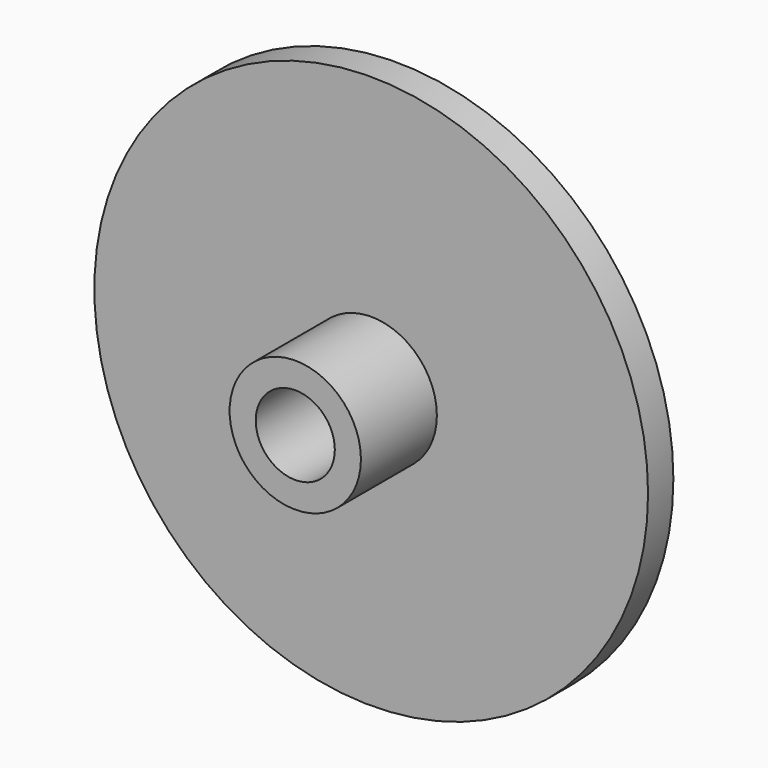
from build123d import *

# Parameters (mm, degrees)
F0_R     = 17.5
F1_DEPTH = 2.00000108
F2_R     = 2.5
F3_DEPTH = 6
F6_DEPTH = 8.00100108
F7_R     = 4.1497915573
F7_R_2   = 2.5
F8_DEPTH = 6


# Not quite as in the source:
# - a feature of the source that left no trace in its solid (it failed there, or was rolled back) is left out
# - a feature names something its author has since deleted; it is built from what else it names
# - the program builds the solid bodies; features that only make, move or delete a surface that nothing else refers to are left out


with BuildPart() as f1:
    # F0 (on Front) → F1 (new body)
    with BuildSketch(Plane.XZ):
        with Locations((-15.6701616943, 19.357258454)):
            Circle(F0_R)
    extrude(amount=F1_DEPTH)

    # F2 (on face) → F3 (join)
    with BuildSketch(Plane.XZ.offset(2.00000108)):
        with Locations((-15.6701616943, 19.357258454)):
            Circle(F2_R)
    extrude(amount=F3_DEPTH)

    # F6 (cut, through all): a face of the model
    f6_faces = [f1.faces().sort_by_distance(p)[0] for p in [
        (-15.6701616943, -8.00000108, 19.357258454),
    ]]
    extrude(f6_faces, amount=-F6_DEPTH, mode=Mode.SUBTRACT)

    # F7 (on face) → F8 (join)
    with BuildSketch(Plane.XZ.offset(2.00000108)):
        with Locations((-15.6701616943, 19.357258454)):
            Circle(F7_R)
        with Locations((-15.6701616943, 19.357258454)):
            Circle(F7_R_2, mode=Mode.SUBTRACT)
    extrude(amount=F8_DEPTH)


solid = f1.part
